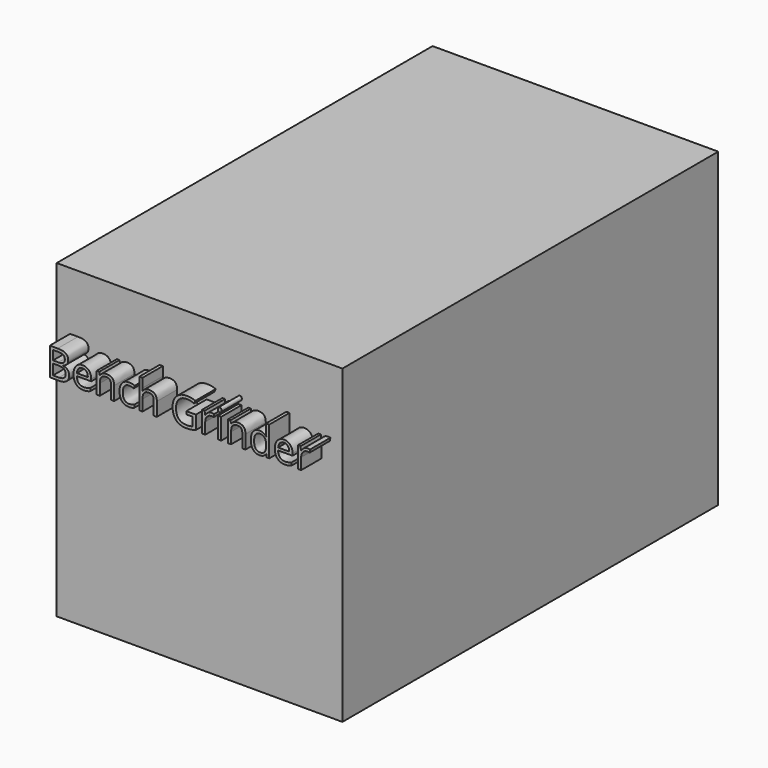
from build123d import *

# Parameters (mm, degrees)
F0_W         = 285.75
F0_H         = 311.15
F1_DEPTH     = 469.9
F2_TEXT_SIZE = 39.1728822895
F3_DEPTH     = 25.4


# Not quite as in the source:
# - Text() gives the source's letters only with a copy of the font that has no kerning and outlines rounded to 1/6400 em; it was checked with that copy


with BuildPart() as f1:
    # F0 (on Front) → F1 (new body)
    with BuildSketch(Plane.XZ):
        Rectangle(F0_W, F0_H)
    extrude(amount=F1_DEPTH)

    # F2 (on face) → F3 (join)
    with BuildSketch(Plane.XZ.offset(469.9)):
        with Locations((-133.35, 69.6007415181)):
            Text('Bench Grinder', F2_TEXT_SIZE, font='Open Sans', text_align=(TextAlign.LEFT, TextAlign.BOTTOM))
    extrude(amount=F3_DEPTH)


solid = f1.part
